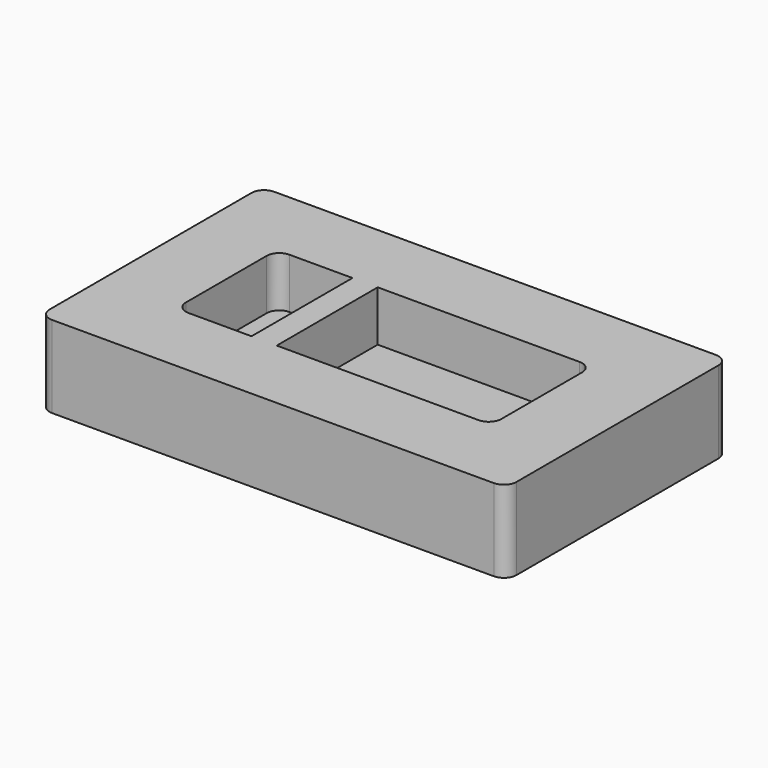
from build123d import *

# Parameters (mm, degrees)
F0_W     = 7.400000114
F0_H     = 4.400000114
F0_W_2   = 5
F0_H_2   = 2
F1_DEPTH = 0.8
F2_DEPTH = 0.5
F4_R     = 0.2
F5_W     = 0.4
F5_H     = 0.8
F6_DEPTH = 2


# Not quite as in the source:
# - a feature names something its author has since deleted; it is built from what else it names


with BuildPart() as f1:
    # F0 (on Top) → F1 (new body)
    with BuildSketch(Plane.XY):
        with Locations((-2.5, -1)):
            Rectangle(F0_W, F0_H)
        with Locations((-2.5, -1)):
            Rectangle(F0_W_2, F0_H_2, mode=Mode.SUBTRACT)
    extrude(amount=F1_DEPTH)

    # F0 (on Top) → F2 (join)
    with BuildSketch(Plane.XY):
        with Locations((-2.5, -1)):
            Rectangle(F0_W, F0_H)
        with Locations((-2.5, -1)):
            Rectangle(F0_W_2, F0_H_2, mode=Mode.SUBTRACT)
        with Locations((-2.5, -1)):
            Rectangle(F0_W_2, F0_H_2)
    extrude(amount=-F2_DEPTH)

    # F4
    f4_edges = [f1.edges().sort_by_distance(p)[0] for p in [
        (-5, 0, 0.4),
        (0, 0, 0.4),
        (0, -2, 0.4),
        (-5, -2, 0.4),
        (-6.2, 1.2, 0.15),
        (1.2, 1.2, 0.15),
        (1.2, -3.2, 0.15),
        (-6.2, -3.2, 0.15),
    ]]
    fillet(f4_edges, radius=F4_R)

    # F5 (on face) → F6 (join, through all)
    with BuildSketch(Plane.XZ):
        with Locations((-3.6, 0.4)):
            Rectangle(F5_W, F5_H)
    extrude(amount=F6_DEPTH)


solid = f1.part
